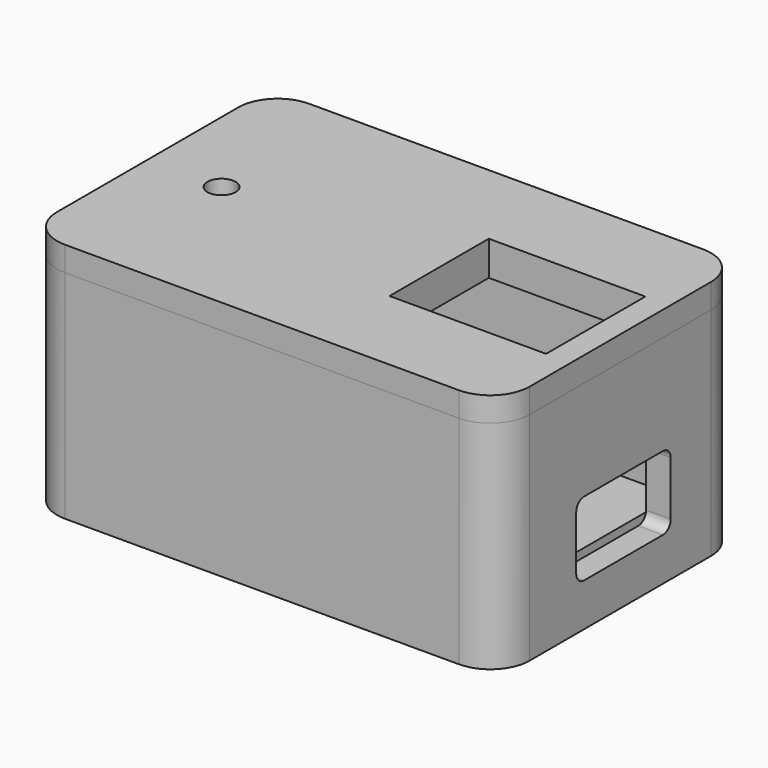
from build123d import *

# Parameters (mm, degrees)
F0_W           = 48
F0_H           = 31
F1_DEPTH       = 22
F2_T           = -2.5
F3_W           = 43
F3_H           = 20
F4_DEPTH       = 2.7
F6_W           = 48
F6_H           = 31
F7_DEPTH       = 2.5
F8_W           = 43
F8_H           = 26.1
F9_DEPTH       = 1
F10_W          = 15.9
F10_H          = 12.6
F11_DEPTH      = 3.5
F12_R          = 4
F12_2_R        = 4
F13_W          = 12
F13_H          = 7.5
F14_DEPTH      = 2.5
F15_T1_DEPTH   = 2.5
F16_R          = 3
F17_DEPTH      = 15.8
F18_R          = 1.425
F19_DEPTH      = 3.5
F19_DEPTH_BACK = 10


# Not quite as in the source:
# - a fillet or chamfer that OpenCascade refuses, or shapes differently, is made with other operations: its cross-section is extruded or revolved along the edge and cut away or added


with BuildPart() as f1:
    # F0 (on Top) → F1 (new body)
    with BuildSketch(Plane.XY):
        Rectangle(F0_W, F0_H)
    extrude(amount=F1_DEPTH)

    # F2
    f2_openings = [f1.faces().sort_by_distance(p)[0] for p in [
        (0, 0, 22),
    ]]
    offset(amount=F2_T, openings=f2_openings)

    # F3 (on face) → F4 (join)
    with BuildSketch(Plane.XY.offset(2.5)):
        Rectangle(F3_W, F3_H)
    extrude(amount=F4_DEPTH)

    # F12
    f12_edges = [f1.edges().sort_by_distance(p)[0] for p in [
        (24, -15.5, 11),
        (-24, -15.5, 11),
        (-24, 15.5, 11),
        (24, 15.5, 11),
    ]]
    fillet(f12_edges, radius=F12_R)

    # F13 (on face) → F14 (cut, through all)
    with BuildSketch(Plane.YZ.offset(24)):
        with Locations((0.3987657316, 8.116890993)):
            Rectangle(F13_W, F13_H)
    extrude(amount=-F14_DEPTH, mode=Mode.SUBTRACT)

    # F15: fillet of radius 1 on 4 edges, made by hand

    # F15_s2 → F15_t1 (join)
    with BuildSketch(Plane.YZ.offset(21.5)):
        with BuildLine():
            ThreePointArc((-4.6012342684, 4.366890993), (-5.3083410496, 4.6597842118), (-5.6012342684, 5.366890993))
            Line((-5.6012342684, 5.366890993), (-5.6012342684, 4.366890993))
            Line((-5.6012342684, 4.366890993), (-4.6012342684, 4.366890993))
        make_face()
        with BuildLine():
            ThreePointArc((6.3987657316, 5.366890993), (6.1058725128, 4.6597842118), (5.3987657316, 4.366890993))
            Line((5.3987657316, 4.366890993), (6.3987657316, 4.366890993))
            Line((6.3987657316, 4.366890993), (6.3987657316, 5.366890993))
        make_face()
        with BuildLine():
            ThreePointArc((6.3987657316, 10.866890993), (6.1058725128, 11.5739977742), (5.3987657316, 11.866890993))
            Line((5.3987657316, 11.866890993), (6.3987657316, 11.866890993))
            Line((6.3987657316, 11.866890993), (6.3987657316, 10.866890993))
        make_face()
        with BuildLine():
            ThreePointArc((-5.6012342684, 10.866890993), (-5.3083410496, 11.5739977742), (-4.6012342684, 11.866890993))
            Line((-4.6012342684, 11.866890993), (-5.6012342684, 11.866890993))
            Line((-5.6012342684, 11.866890993), (-5.6012342684, 10.866890993))
        make_face()
    extrude(amount=F15_T1_DEPTH)

    # F16 (on face) → F17 (join, through all)
    with BuildSketch(Plane.XY.offset(5.2)):
        with Locations((-16.4979076515, 0)):
            Circle(F16_R)
    extrude(amount=F17_DEPTH)


with BuildPart() as f7:
    # F6 (on offset) → F7 (new body)
    with BuildSketch(Plane.XY.offset(24.5)):
        Rectangle(F6_W, F6_H)
    extrude(amount=-F7_DEPTH)

    # F8 (on face) → F9 (join)
    with BuildSketch(Plane(origin=(0, 0, 22), x_dir=(1, 0, 0), z_dir=(0, 0, -1))):
        Rectangle(F8_W, F8_H)
    extrude(amount=F9_DEPTH)

    # F10 (on face) → F11 (cut, through all)
    with BuildSketch(Plane(origin=(0, 0, 21), x_dir=(1, 0, 0), z_dir=(0, 0, -1))):
        with Locations((13.55, 0)):
            Rectangle(F10_W, F10_H)
    extrude(amount=-F11_DEPTH, mode=Mode.SUBTRACT)

    # F12#2
    f12_2_edges = [f7.edges().sort_by_distance(p)[0] for p in [
        (24, -15.5, 23.25),
        (24, 15.5, 23.25),
        (-24, -15.5, 23.25),
        (-24, 15.5, 23.25),
    ]]
    fillet(f12_2_edges, radius=F12_2_R)


with BuildPart() as f19_tool:
    # F18 (on face) → F19 (new body, two sides)
    with BuildSketch(Plane.XY.offset(21)) as f19_sk:
        with Locations((-16.4979076515, 0)):
            Circle(F18_R)
    extrude(amount=F19_DEPTH)
    extrude(f19_sk.sketch, amount=-F19_DEPTH_BACK)


with BuildPart() as f1_1:
    add(f1.part)

    # F19: cut by f19_tool
    add(f19_tool.part, mode=Mode.SUBTRACT)


with BuildPart() as f7_1:
    add(f7.part)

    # F19: cut by f19_tool
    add(f19_tool.part, mode=Mode.SUBTRACT)


solid = Compound([f1_1.part, f7_1.part])
